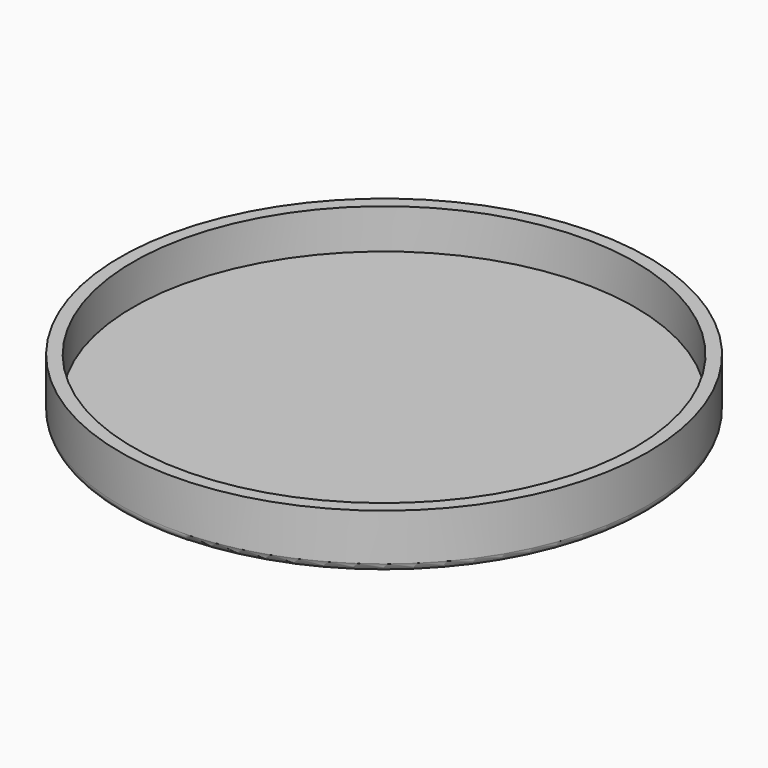
from build123d import *

# Parameters (mm, degrees)
F0_R         = 53
F1_DEPTH     = 3
F2_R         = 53
F2_R_2       = 50.4
F3_DEPTH     = 8
F4_TEXT_SIZE = 11.4744973583
F5_DEPTH     = 1.2
F6_R         = 1.6


# Not quite as in the source:
# - Text() gives the source's letters only with a copy of the font that has no kerning and outlines rounded to 1/6400 em; it was checked with that copy


with BuildPart() as f1:
    # F0 (on Top) → F1 (new body)
    with BuildSketch(Plane.XY):
        Circle(F0_R)
    extrude(amount=F1_DEPTH)

    # F2 (on face) → F3 (join)
    with BuildSketch(Plane.XY.offset(3)):
        Circle(F2_R)
        Circle(F2_R_2, mode=Mode.SUBTRACT)
    extrude(amount=F3_DEPTH)

    # F4 (on face) → F5 (cut)
    with BuildSketch(Plane(origin=(0, 0, 0), x_dir=(1, 0, 0), z_dir=(0, 0, -1))):
        with Locations((-32.9000093043, -3.6999997683)):
            Text('Apo-Nikkor', F4_TEXT_SIZE, font='Open Sans', font_style=FontStyle.BOLD, text_align=(TextAlign.LEFT, TextAlign.BOTTOM))
    extrude(amount=-F5_DEPTH, mode=Mode.SUBTRACT)

    # F6
    f6_edges = [f1.edges().sort_by_distance(p)[0] for p in [
        (-53, 0, 0),
    ]]
    fillet(f6_edges, radius=F6_R)


solid = f1.part
